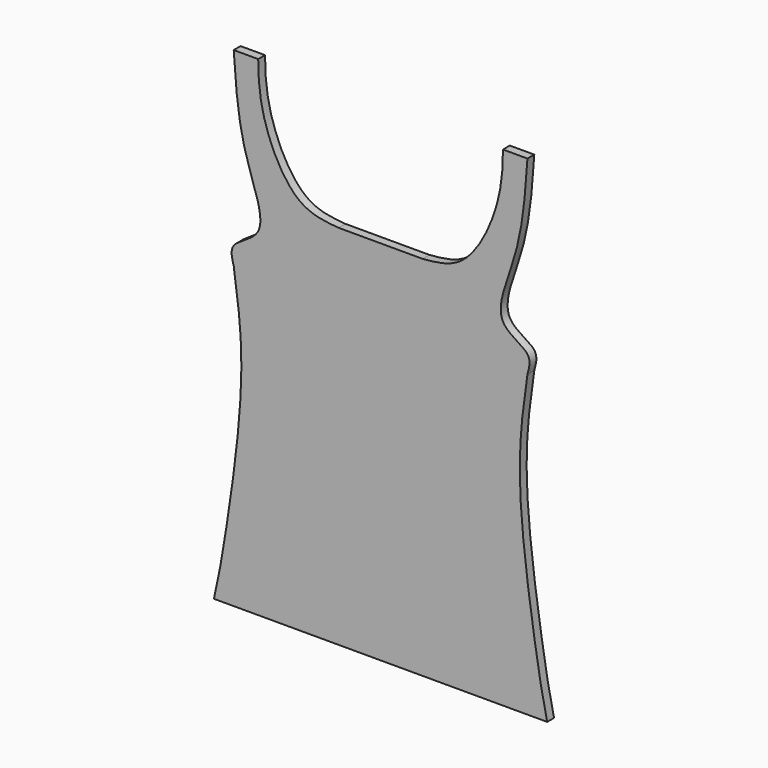
from build123d import *

# Parameters (mm, degrees)
F1_DEPTH = 8.89


with BuildPart() as f1:
    # F0 (on Front) → F1 (new body)
    with BuildSketch(Plane.XZ):
        with BuildLine():
            Line((152.4, 0), (127, 0))
            add(Edge.make_bspline(
                [(127, 0), (127, -20.0168341398), (123.3922770096, -58.2410161724), (89.3160713506, -123.1038827606), (57.5735042432, -125.7764468865), (43.5800775886, -127)],
                knots=[0, 0, 0, 0, 0.345812323, 0.7105558481, 1, 1, 1, 1], degree=3))
            Line((43.5800775886, -127), (0, -127))
            Line((0, -127), (-43.5800775886, -127))
            add(Edge.make_bspline(
                [(-127, 0), (-127, -20.0168341398), (-123.3922770096, -58.2410161724), (-89.3160713506, -123.1038827606), (-57.5735042432, -125.7764468865), (-43.5800775886, -127)],
                knots=[0, 0, 0, 0, 0.345812323, 0.7105558481, 1, 1, 1, 1], degree=3))
            Line((-127, 0), (-152.4, 0))
            add(Edge.make_bspline(
                [(-152.4, 0), (-150.2703878505, -31.3639571024), (-146.3939702155, -88.3715453558), (-110.9714635835, -160.9462971944), (-158.6767490389, -174.9726116512), (-154.2449504284, -190.6305366091), (-152.4, -197.1800625324)],
                knots=[0, 0, 0, 0, 0.3476574396, 0.6384459753, 0.8455987873, 1, 1, 1, 1], degree=3))
            add(Edge.make_bspline(
                [(-152.4, -197.1800625324), (-148.2010351465, -226.5358633988), (-138.5263708492, -292.0003756963), (-159.3646682678, -437.8166234112), (-168.1102758726, -487.6635444085), (-172.8998571634, -508)],
                knots=[0, 0, 0, 0, 0.3238760373, 0.7228207872, 1, 1, 1, 1], degree=3))
            Line((-172.8998571634, -508), (0, -508))
            Line((0, -508), (172.8998571634, -508))
            add(Edge.make_bspline(
                [(152.4, -197.1800625324), (148.2010351465, -226.5358633988), (138.5263708492, -292.0003756963), (159.3646682678, -437.8166234112), (168.1102758726, -487.6635444085), (172.8998571634, -508)],
                knots=[0, 0, 0, 0, 0.3238760373, 0.7228207872, 1, 1, 1, 1], degree=3))
            add(Edge.make_bspline(
                [(152.4, 0), (150.2703878505, -31.3639571024), (146.3939702155, -88.3715453558), (110.9714635835, -160.9462971944), (158.6767490389, -174.9726116512), (154.2449504284, -190.6305366091), (152.4, -197.1800625324)],
                knots=[0, 0, 0, 0, 0.3476574396, 0.6384459753, 0.8455987873, 1, 1, 1, 1], degree=3))
        make_face()
    extrude(amount=F1_DEPTH)


solid = f1.part
